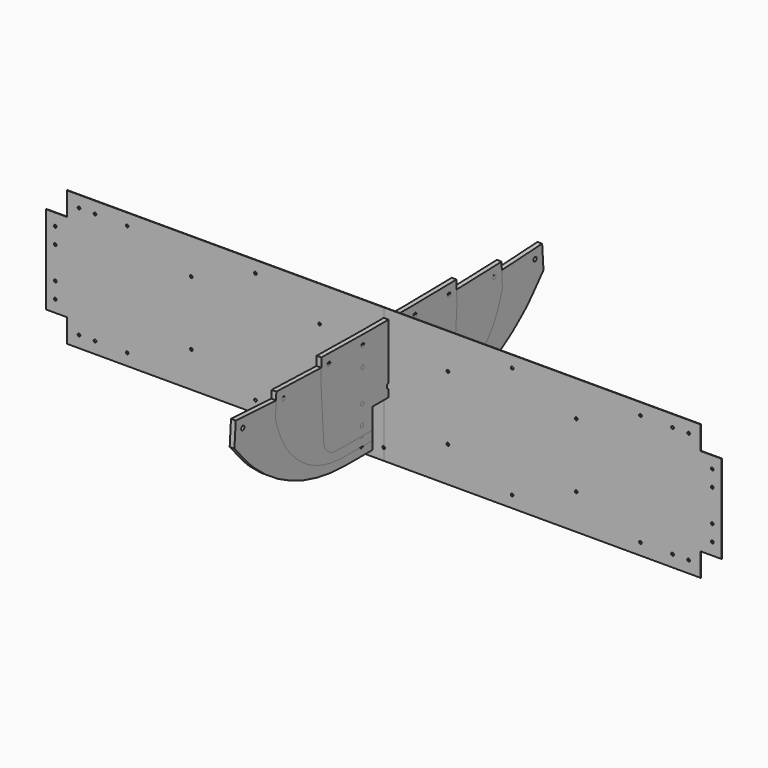
from build123d import *
from build123d import SkipClean  # not in build123d's __all__

# Parameters (mm, degrees)
F3_R      = 2
F11_DEPTH = 0.8
F12_DEPTH = 0.8
F4_R      = 3
F4_R_2    = 4
F15_DEPTH = 7
F7_R      = 3
F7_R_2    = 4
F10_R     = 3
F10_R_2   = 4


with BuildPart() as f11:
    # F3 (on Front) → F11 (new body)
    with BuildSketch(Plane.XZ):
        with BuildLine():
            Line((0, 100), (-469.1, 100))
            Line((-469.1, 100), (-469.1, 65.35))
            Line((-469.1, 65.35), (-500, 65.35))
            Line((-500, 65.35), (-500, 0))
            Line((-500, 0), (0, 0))
            Line((0, 0), (0, 80.675))
            ThreePointArc((0, 80.675), (-2, 82.675), (0, 84.675))
            Line((0, 84.675), (0, 100))
        make_face()
        with Locations((-486.425, 23.75)):
            Circle(F3_R, mode=Mode.SUBTRACT)
        with Locations((-486.425, 47.5)):
            Circle(F3_R, mode=Mode.SUBTRACT)
        with Locations((-285, 47.5)):
            Circle(F3_R, mode=Mode.SUBTRACT)
        with Locations((-95, 47.5)):
            Circle(F3_R, mode=Mode.SUBTRACT)
        with Locations((-451.25, 82.675)):
            Circle(F3_R, mode=Mode.SUBTRACT)
        with Locations((-427.5, 82.675)):
            Circle(F3_R, mode=Mode.SUBTRACT)
        with Locations((-380, 82.675)):
            Circle(F3_R, mode=Mode.SUBTRACT)
        with Locations((-190, 82.675)):
            Circle(F3_R, mode=Mode.SUBTRACT)
        with BuildLine():
            Line((0, 80.675), (0, 84.675))
            ThreePointArc((0, 84.675), (-2, 82.675), (0, 80.675))
        make_face()
    extrude(amount=F11_DEPTH)

    # F3 (on Front) → F12 (cut)
    with BuildSketch(Plane.XZ):
        with BuildLine():
            Line((0, 80.675), (0, 84.675))
            ThreePointArc((0, 84.675), (-2, 82.675), (0, 80.675))
        make_face()
    extrude(amount=F12_DEPTH, mode=Mode.SUBTRACT)

    # F13: F11 across plane


with BuildPart() as f11_1:
    add(f11.part, clean=False)
    add(f11.part.mirror(Plane.XY), clean=False)

    # F14: F11 across plane


with BuildPart() as f11_2:
    add(f11_1.part, clean=False)
    with SkipClean():  # cleaning this boolean's faces spoils the solid; the shape is the same uncleaned
        add(f11_1.part.mirror(Plane.YZ), clean=False)


with BuildPart() as f15:
    # F4 (on Right) → F15 (new body)
    with BuildSketch(Plane.YZ):
        with BuildLine():
            ThreePointArc((283.5459854903, 69.7853243935), (0, 60), (-283.5459854903, 69.7853243935))
            Line((-283.5459854904, 69.7853243935), (-286.0071067357, 34.1702590108))
            Line((-286.0071067357, 34.1702590108), (-266.5469280434, 11.8209001342))
            ThreePointArc((-266.5469280434, 11.8209001342), (-257.7634411548, 2.3132281924), (-248.4360051401, -6.6614252866))
            ThreePointArc((-248.4360051401, -6.6614252866), (-170.4931430202, -54.7200262189), (-80.4736738133, -71.489463977))
            Line((-80.4736738133, -71.489463977), (-30, -71.489463977))
            Line((-30, -71.489463977), (-30, -15))
            Line((-30, -15), (30, -15))
            Line((30, -15), (30, -71.489463977))
            Line((30, -71.489463977), (80.4736738133, -71.489463977))
            ThreePointArc((80.4736738133, -71.489463977), (170.4931430202, -54.7200262189), (248.4360051401, -6.6614252866))
            ThreePointArc((248.4360051401, -6.6614252866), (257.7634411547, 2.3132281923), (266.5469280434, 11.8209001342))
            Line((266.5469280434, 11.8209001342), (286.0071067357, 34.1702590108))
            Line((286.0071067357, 34.1702590108), (283.5459854904, 69.7853243935))
        make_face()
        with Locations((-50.582221288, -58.0395296416)):
            Circle(F4_R, mode=Mode.SUBTRACT)
        with Locations((-50.0122002711, -29.7452709299)):
            Circle(F4_R, mode=Mode.SUBTRACT)
        with Locations((50.582221288, -58.0395296416)):
            Circle(F4_R, mode=Mode.SUBTRACT)
        with Locations((50.0122002711, -29.7452709299)):
            Circle(F4_R, mode=Mode.SUBTRACT)
        Circle(F4_R_2, mode=Mode.SUBTRACT)
        with Locations((-49.0554512144, 17.745092632)):
            Circle(F4_R, mode=Mode.SUBTRACT)
        with Locations((-183.8780596918, 49.9982695657)):
            Circle(F4_R, mode=Mode.SUBTRACT)
        with Locations((-270.4499306435, 54.77086055)):
            Circle(F4_R, mode=Mode.SUBTRACT)
        with Locations((-48.4854301975, 46.0393513436)):
            Circle(F4_R, mode=Mode.SUBTRACT)
        with Locations((49.0554512144, 17.745092632)):
            Circle(F4_R, mode=Mode.SUBTRACT)
        with Locations((48.4854301975, 46.0393513436)):
            Circle(F4_R, mode=Mode.SUBTRACT)
        with Locations((183.8780596918, 49.9982695657)):
            Circle(F4_R, mode=Mode.SUBTRACT)
        with Locations((270.4499306435, 54.77086055)):
            Circle(F4_R, mode=Mode.SUBTRACT)
    extrude(amount=F15_DEPTH)


with BuildPart() as f15b:
    # F7 (on Right) → F15, piece 2 (new body)
    with BuildSketch(Plane.YZ):
        with BuildLine():
            ThreePointArc((208.4388718574, 76.9179450014), (0, 72.546), (-208.4388718574, 76.9179450014))
            Line((-208.4388718574, 76.9179450014), (-209.9358076299, 41.249342796))
            Line((-209.9358076299, 41.249342796), (-205.8019202456, 28.2151746717))
            ThreePointArc((-205.8019202456, 28.2151746717), (-161.4808508573, -34.1225678307), (-89.1418005751, -58.9703672559))
            ThreePointArc((-89.1418005751, -58.9703672559), (-76.6424210945, -59.1571947346), (-64.1418005751, -59.2194726218))
            Line((-64.1418005751, -59.2194726218), (-30, -59.2194726218))
            Line((-30, -59.2194726218), (-30, -15))
            Line((-30, -15), (30, -15))
            Line((30, -15), (30, -59.2194726218))
            Line((30, -59.2194726218), (64.1418005751, -59.2194726218))
            ThreePointArc((64.1418005751, -59.2194726218), (76.6424210945, -59.1571947346), (89.1418005751, -58.9703672559))
            ThreePointArc((89.1418005751, -58.9703672559), (161.4808508573, -34.1225678307), (205.8019202456, 28.2151746717))
            Line((205.8019202456, 28.2151746717), (209.9358076299, 41.249342796))
            Line((209.9358076299, 41.249342796), (208.4388718574, 76.9179450014))
        make_face()
        with Locations((-50.1708855913, -45.5246562927)):
            Circle(F7_R, mode=Mode.SUBTRACT)
        with Locations((-49.6992407607, -17.2285867572)):
            Circle(F7_R, mode=Mode.SUBTRACT)
        Circle(F7_R_2, mode=Mode.SUBTRACT)
        with Locations((50.1708855913, -45.5246562927)):
            Circle(F7_R, mode=Mode.SUBTRACT)
        with Locations((49.6992407607, -17.2285867572)):
            Circle(F7_R, mode=Mode.SUBTRACT)
        with Locations((-48.9076107448, 30.2648161733)):
            Circle(F7_R, mode=Mode.SUBTRACT)
        with Locations((-194.941677367, 62.2590425536)):
            Circle(F7_R, mode=Mode.SUBTRACT)
        with Locations((-48.4359659142, 58.5608857087)):
            Circle(F7_R, mode=Mode.SUBTRACT)
        with Locations((48.9076107448, 30.2648161733)):
            Circle(F7_R, mode=Mode.SUBTRACT)
        with Locations((48.4359659142, 58.5608857087)):
            Circle(F7_R, mode=Mode.SUBTRACT)
        with Locations((194.941677367, 62.2590425536)):
            Circle(F7_R, mode=Mode.SUBTRACT)
    extrude(amount=F15_DEPTH)


with BuildPart() as f15c:
    # F10 (on Right) → F15, piece 3 (new body)
    with BuildSketch(Plane.YZ):
        with BuildLine():
            ThreePointArc((124.9909156074, 87.5410812079), (0, 86.236), (-124.9909156074, 87.5410812079))
            Line((-124.9909156074, 87.5410812079), (-125.7363509043, 51.8488646024))
            Line((-125.7363509043, 51.8488646024), (-120.6483548376, -24.6829629057))
            ThreePointArc((-120.6483548376, -24.6829629057), (-113.9039304957, -39.1214893804), (-99.1802213367, -45.2182668132))
            ThreePointArc((-99.1802213367, -45.2182668132), (-79.5912932248, -45.5411443506), (-60, -45.6487745275))
            Line((-60, -45.6487745275), (-30, -45.6487745275))
            Line((-30, -45.6487745275), (-30, -15))
            Line((-30, -15), (30, -15))
            Line((30, -15), (30, -45.6487745275))
            Line((30, -45.6487745275), (60, -45.6487745275))
            ThreePointArc((60, -45.6487745275), (79.5912932248, -45.5411443506), (99.1802213367, -45.2182668132))
            ThreePointArc((99.1802213367, -45.2182668132), (113.9039304957, -39.1214893804), (120.6483548376, -24.6829629057))
            Line((120.6483548376, -24.6829629057), (125.7363509043, 51.8488646024))
            Line((125.7363509043, 51.8488646024), (124.9909156074, 87.5410812079))
        make_face()
        with Locations((-49.8365836496, -31.8589023938)):
            Circle(F10_R, mode=Mode.SUBTRACT)
        with Locations((-49.4449063789, -3.5616129668)):
            Circle(F10_R, mode=Mode.SUBTRACT)
        Circle(F10_R_2, mode=Mode.SUBTRACT)
        with Locations((49.8365836496, -31.8589023938)):
            Circle(F10_R, mode=Mode.SUBTRACT)
        with Locations((49.4449063789, -3.5616129668)):
            Circle(F10_R, mode=Mode.SUBTRACT)
        with Locations((-48.7874975323, 43.9338374849)):
            Circle(F10_R, mode=Mode.SUBTRACT)
        with Locations((-111.188069141, 73.1663035153)):
            Circle(F10_R, mode=Mode.SUBTRACT)
        with Locations((-48.3958202616, 72.2311269119)):
            Circle(F10_R, mode=Mode.SUBTRACT)
        with Locations((48.7874975323, 43.9338374849)):
            Circle(F10_R, mode=Mode.SUBTRACT)
        with Locations((48.3958202616, 72.2311269119)):
            Circle(F10_R, mode=Mode.SUBTRACT)
        with Locations((111.188069141, 73.1663035153)):
            Circle(F10_R, mode=Mode.SUBTRACT)
    extrude(amount=F15_DEPTH)


solid = Compound([f11_2.part, f15.part, f15b.part, f15c.part])
